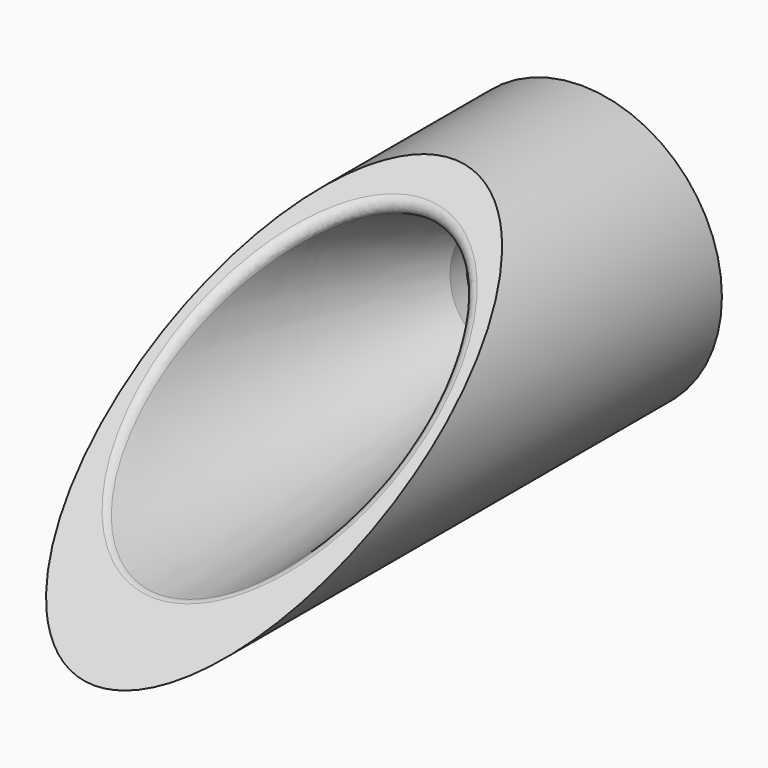
from build123d import *

# Parameters (mm, degrees)
F0_R     = 14.6
F1_DEPTH = 65
F6_W     = 44.992752164
F6_H     = 26.5233175738
F7_DEPTH = 77.8942202739
F10_R    = 1


with BuildPart() as f1:
    # F0 (on Front) → F1 (new body)
    with BuildSketch(Plane.XZ):
        Circle(F0_R)
    extrude(amount=-F1_DEPTH)

    # F6 (on face) → F7 (cut, through all)
    with BuildSketch(Plane(origin=(-1.2201803985, -11.8274942396, -7.3906386602), x_dir=(0.9961946981, -0.0739122617, -0.0461855071), z_dir=(-0.0871557427, -0.8448210171, -0.5279027614))):
        Rectangle(F6_W, F6_H)
    extrude(amount=-F7_DEPTH, mode=Mode.SUBTRACT)

    # F8 (on Right) → F9 (revolve, cut)
    with BuildSketch(Plane.YZ):
        with BuildLine():
            Line((65, -3.9643939246), (65.3479595253, -1.3373377453))
            Line((65.3479595253, -1.3373377453), (55.2512065056, 0))
            Line((55.2512065056, 0), (11.6982164167, 5.7686919206))
            Line((11.6982164167, 5.7686919206), (9.6625984549, -9.6))
            ThreePointArc((9.6625984549, -9.6), (32.15326072, -8.6481356715), (54.4830694403, -5.7993504334))
            Line((54.4830694403, -5.7993504334), (56.6640217401, -6.0882224921))
            Line((56.6640217401, -6.0882224921), (60.0792311345, -4.6744174164))
            Line((60.0792311345, -4.6744174164), (61, -3.4345848888))
            Line((61, -3.4345848888), (65, -3.9643939246))
        make_face()
    revolve(axis=Axis((0, 47.6560502276, 1.005995606), (0, 0.9913419544, -0.1313054812)), mode=Mode.SUBTRACT)

    # F10
    f10_edges = [f1.edges().sort_by_distance(p)[0] for p in [
        (0, 43.159876, 11.331422),
    ]]
    fillet(f10_edges, radius=F10_R)


solid = f1.part
